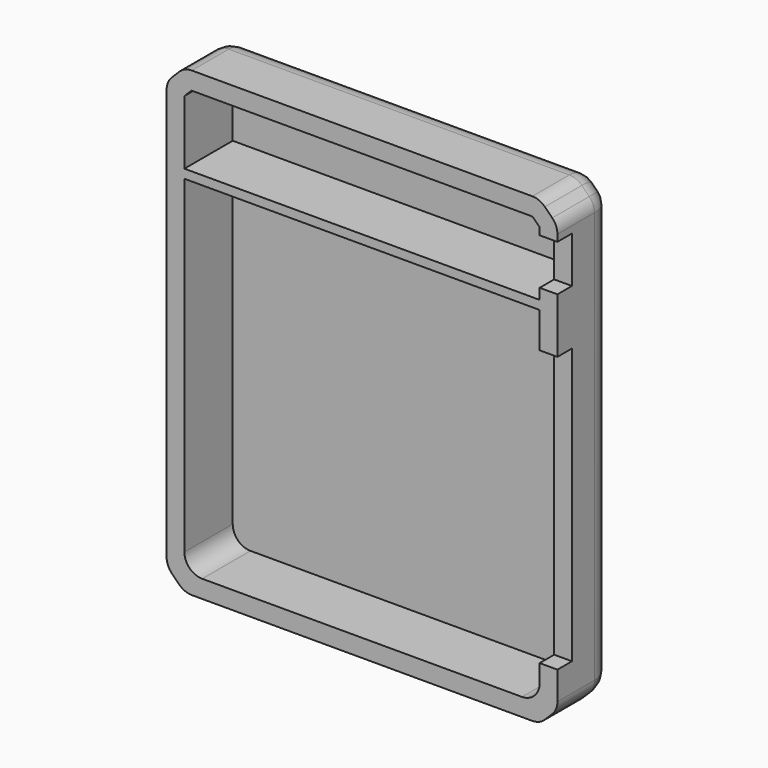
from build123d import *

# Parameters (mm, degrees)
F0_W      = 110
F0_H      = 130
F1_DEPTH  = 20
F2_W      = 100
F2_H      = 120
F3_DEPTH  = 17
F4_W      = 100
F4_H      = 2.5
F5_DEPTH  = 17
F6_SIZE   = 5
F7_SIZE   = 2
F8_R      = 7
F9_R      = 5
F10_R     = 5
F11_R     = 5
F12_W     = 5
F12_H     = 77.5
F13_DEPTH = 5.1
F14_W     = 5
F14_H     = 13
F15_DEPTH = 5.1


with BuildPart() as f1:
    # F0 (on Front) → F1 (new body)
    with BuildSketch(Plane.XZ):
        Rectangle(F0_W, F0_H)
    extrude(amount=F1_DEPTH)

    # F2 (on face) → F3 (cut)
    with BuildSketch(Plane.XZ.offset(20)):
        Rectangle(F2_W, F2_H)
    extrude(amount=-F3_DEPTH, mode=Mode.SUBTRACT)

    # F4 (on face) → F5 (join, through all)
    with BuildSketch(Plane.XZ.offset(3)):
        with Locations((0, 38.75)):
            Rectangle(F4_W, F4_H)
    extrude(amount=F5_DEPTH)

    # F6
    f6_edges = [f1.edges().sort_by_distance(p)[0] for p in [
        (55, -10, 65),
        (-55, -10, 65),
        (55, -10, -65),
        (-55, -10, -65),
    ]]
    chamfer(f6_edges, length=F6_SIZE)

    # F7
    f7_edges = [f1.edges().sort_by_distance(p)[0] for p in [
        (50, -11.5, 60),
        (-50, -11.5, 60),
    ]]
    chamfer(f7_edges, length=F7_SIZE)

    # F8
    f8_edges = [f1.edges().sort_by_distance(p)[0] for p in [
        (0, 0, -65),
        (-52.5, 0, -62.5),
        (52.5, 0, -62.5),
        (-55, 0, 0),
        (55, 0, 0),
        (-52.5, 0, 62.5),
        (52.5, 0, 62.5),
        (0, 0, 65),
    ]]
    fillet(f8_edges, radius=F8_R)

    # F9
    f9_edges = [f1.edges().sort_by_distance(p)[0] for p in [
        (-55, -13.5, -60),
        (-50, -13.5, -65),
        (55, -13.5, -60),
        (50, -13.5, -65),
        (50, -13.5, 65),
        (55, -13.5, 60),
    ]]
    fillet(f9_edges, radius=F9_R)

    # F10
    f10_edges = [f1.edges().sort_by_distance(p)[0] for p in [
        (-50, -13.5, 65),
        (-55, -13.5, 60),
    ]]
    fillet(f10_edges, radius=F10_R)

    # F11
    f11_edges = [f1.edges().sort_by_distance(p)[0] for p in [
        (-50, -11.5, -60),
        (50, -11.5, -60),
    ]]
    fillet(f11_edges, radius=F11_R)

    # F12 (on face) → F13 (cut)
    with BuildSketch(Plane.XZ.offset(20)):
        with Locations((52.5, -11.25)):
            Rectangle(F12_W, F12_H)
    extrude(amount=-F13_DEPTH, mode=Mode.SUBTRACT)

    # F14 (on face) → F15 (cut)
    with BuildSketch(Plane.XZ.offset(20)):
        with Locations((52.5, 49.5)):
            Rectangle(F14_W, F14_H)
    extrude(amount=-F15_DEPTH, mode=Mode.SUBTRACT)


solid = f1.part
